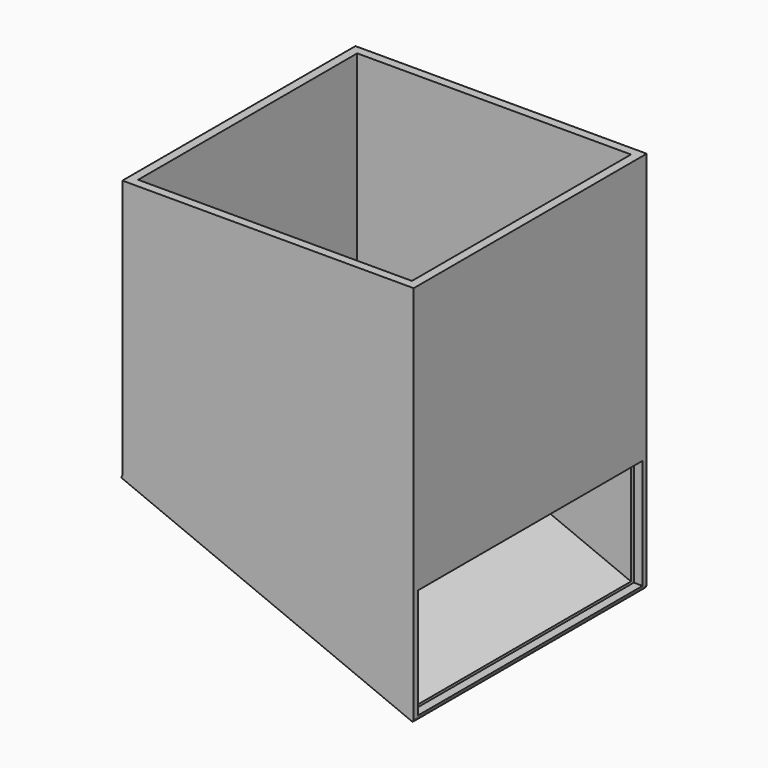
from build123d import *

# Parameters (mm, degrees)
F0_W      = 127
F0_H      = 127
F0_W_2    = 119.38
F0_H_2    = 119.38
F1_DEPTH  = 177.8
F10_DEPTH = 127.001
F11_W     = 137.4053613401
F11_H     = 127
F12_DEPTH = 1.27
F13_W     = 122.4279999733
F13_H     = 48.0059999866
F14_DEPTH = 3.81


# Not quite as in the source:
# - a feature of the source that left no trace in its solid (it failed there, or was rolled back) is left out
# - a feature names something its author has since deleted; it is built from what else it names


with BuildPart() as f1:
    # F0 (on Top) → F1 (new body)
    with BuildSketch(Plane.XY):
        Rectangle(F0_W, F0_H)
        Rectangle(F0_W_2, F0_H_2, mode=Mode.SUBTRACT)
    extrude(amount=F1_DEPTH)

    # F8: union 

    # F9 (on face) → F10 (cut, through all)
    with BuildSketch(Plane.XZ.offset(63.5)):
        Polygon((75.6702050567, -13.2453246042), (93.3672711253, 0), (-89.8822396994, 75.6837800145), (-89.8822396994, -21.479823067), align=None)
    extrude(amount=-F10_DEPTH, mode=Mode.SUBTRACT)

    # F11 (on face) → F12 (join)
    with BuildSketch(Plane(origin=(13.6055070593, 0, 32.9423624542), x_dir=(0.924272523, 0, -0.3817332881), z_dir=(-0.3817332881, 0, -0.924272523))):
        with Locations((-14.7202331787, 0)):
            Rectangle(F11_W, F11_H)
    extrude(amount=F12_DEPTH)

    # F13 (on face) → F14 (cut)
    with BuildSketch(Plane.YZ.offset(63.5)):
        with Locations((0, 36.8464652686)):
            Rectangle(F13_W, F13_H)
    extrude(amount=-F14_DEPTH, mode=Mode.SUBTRACT)


solid = f1.part
